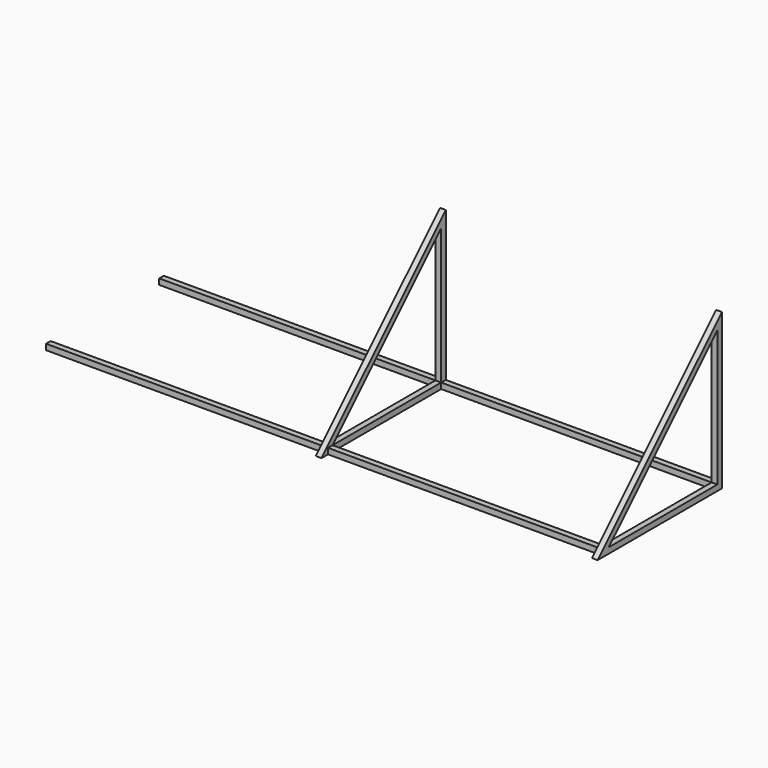
from build123d import *

# Parameters (mm, degrees)
F1_DEPTH = 25.4
F2_W     = 25.4
F2_H     = 25.4
F3_DEPTH = 1219.2


with BuildPart() as f1:
    # F0 (on Right) → F1 (new body)
    with BuildSketch(Plane.YZ):
        Polygon((-685.8, 0), (0, 0), (0, 685.8), align=None)
        Polygon((-25.4, 624.4789755157), (-25.4, 25.4), (-624.4789755157, 25.4), align=None, mode=Mode.SUBTRACT)
    extrude(amount=F1_DEPTH)

    # F2 (on face) → F3 (join)
    with BuildSketch(Plane(origin=(0, 0, 0), x_dir=(0, -1, 0), z_dir=(-1, 0, 0))):
        with Locations((12.7, 12.7)):
            Rectangle(F2_W, F2_H)
        with Locations((637.1789755157, 12.7)):
            Rectangle(F2_W, F2_H)
    extrude(amount=F3_DEPTH)


with BuildPart() as f4_1:
    # F4: copy of F1
    add(f1.part.moved(Location((1219.2, 0, 0))))


solid = Compound([f1.part, f4_1.part])
